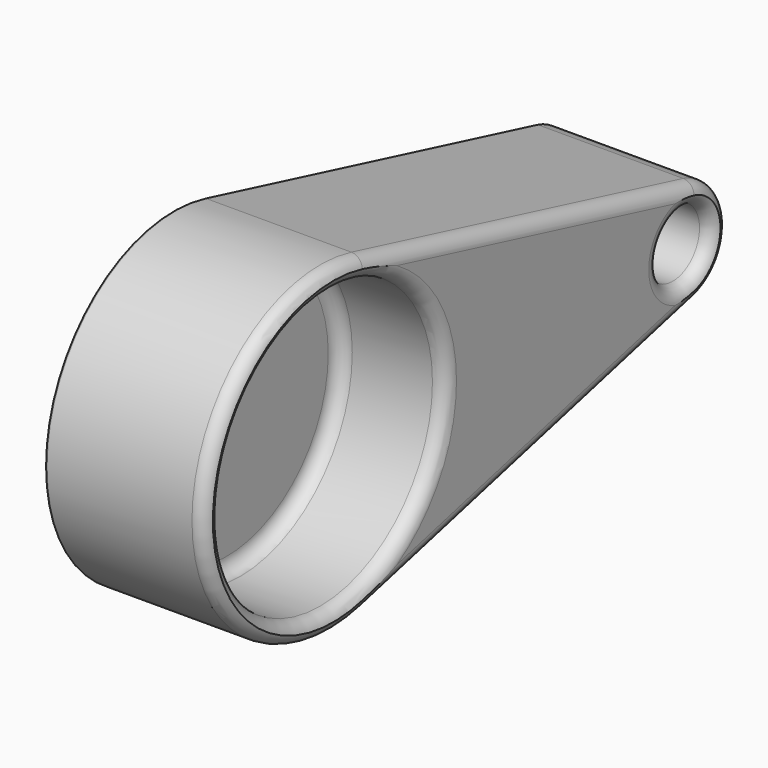
from build123d import *

# Parameters (mm, degrees)
F1_DEPTH = 76.2
F2_R     = 66.675
F2_R_2   = 15.875
F3_DEPTH = 50.8
F4_F1_R  = 6.35
F4_F2_R  = 6.35
F4_F3_R  = 6.35
F5_T     = -2.54
F6_R     = 1


# Not quite as in the source:
# - a fillet or chamfer that OpenCascade refuses, or shapes differently, is made with other operations: its cross-section is extruded or revolved along the edge and cut away or added


with BuildPart() as f1:
    # F0 (on Right) → F1 (new body)
    with BuildSketch(Plane.YZ):
        with BuildLine():
            ThreePointArc((18.4812146278, -73.9248585111), (60.0612543768, -46.8944103565), (76.2, 0))
            ThreePointArc((76.2, 0), (60.0612543768, 46.8944103565), (18.4812146278, 73.9248585111))
            ThreePointArc((18.4812146278, 73.9248585111), (-76.2, 0), (18.4812146278, -73.9248585111))
        make_face()
        with BuildLine():
            ThreePointArc((18.4812146278, 73.9248585111), (60.0612543768, 46.8944103565), (76.2, 0))
            ThreePointArc((76.2, 0), (60.0612543768, -46.8944103565), (18.4812146278, -73.9248585111))
            Line((18.4812146278, -73.9248585111), (215.6141706573, -24.6416195037))
            ThreePointArc((215.6141706573, -24.6416195037), (184.0537657814, 0), (215.6141706573, 24.6416195037))
            Line((215.6141706573, 24.6416195037), (18.4812146278, 73.9248585111))
        make_face()
        with BuildLine():
            ThreePointArc((234.8537657814, 0), (229.474183907, 15.6314701188), (215.6141706573, 24.6416195037))
            ThreePointArc((215.6141706573, 24.6416195037), (184.0537657814, 0), (215.6141706573, -24.6416195037))
            ThreePointArc((215.6141706573, -24.6416195037), (229.474183907, -15.6314701188), (234.8537657814, 0))
        make_face()
    extrude(amount=F1_DEPTH)

    # F2 (on face) → F3 (cut)
    with BuildSketch(Plane.YZ.offset(76.2)):
        Circle(F2_R)
        with Locations((209.4537657814, 0)):
            Circle(F2_R_2)
    extrude(amount=-F3_DEPTH, mode=Mode.SUBTRACT)

    # F4: fillet of radius 6.35 on 8 edges, made by hand

    # F4_f1
    f4_f1_edges = [f1.edges().sort_by_distance(p)[0] for p in [
        (76.2, -76.2, 0),
        (76.2, 117.0476926425, 49.2832390074),
        (76.2, 117.0476926425, -49.2832390074),
        (76.2, 234.8537657814, 0),
    ]]
    fillet(f4_f1_edges, radius=F4_F1_R)

    # F4_f2
    f4_f2_edges = [f1.edges().sort_by_distance(p)[0] for p in [
        (25.4, -66.675, 0),
    ]]
    fillet(f4_f2_edges, radius=F4_F2_R)

    # F4_f3
    f4_f3_edges = [f1.edges().sort_by_distance(p)[0] for p in [
        (25.4, 193.5787657814, 0),
    ]]
    fillet(f4_f3_edges, radius=F4_F3_R)

    # F4_s4 → F4_t5 (revolve, cut)
    with BuildSketch(Plane.XY):
        with BuildLine():
            ThreePointArc((76.2, 73.025), (74.3401280605, 68.5348719395), (69.85, 66.675))
            Line((69.85, 66.675), (69.85, 66.548))
            Line((69.85, 66.548), (76.327, 66.548))
            Line((76.327, 66.548), (76.327, 73.025))
            Line((76.327, 73.025), (76.2, 73.025))
        make_face()
    revolve(axis=Axis((76.2, 0, 0), (1, 0, 0)), mode=Mode.SUBTRACT)

    # F4_s6 → F4_t7 (revolve, cut)
    with BuildSketch(Plane.XY):
        with BuildLine():
            ThreePointArc((69.85, 225.3287657814), (74.3401280605, 227.1886377208), (76.2, 231.6787657814))
            Line((76.2, 231.6787657814), (76.327, 231.6787657814))
            Line((76.327, 231.6787657814), (76.327, 225.2017657814))
            Line((76.327, 225.2017657814), (69.85, 225.2017657814))
            Line((69.85, 225.2017657814), (69.85, 225.3287657814))
        make_face()
    revolve(axis=Axis((76.2, 209.4537657814, 0), (1, 0, 0)), mode=Mode.SUBTRACT)

    # F5
    f5_openings = [f1.faces().sort_by_distance(p)[0] for p in [
        (0, 57.51924, 0),
    ]]
    offset(amount=F5_T, openings=f5_openings)

    # F6
    f6_edges = [f1.edges().sort_by_distance(p)[0] for p in [
        (0, 117.047693, -49.283239),
        (0, 116.431652, -46.819077),
        (0, -76.2, 0),
        (0, -73.66, 0),
        (0, 116.431652, 46.819077),
        (0, 117.047693, 49.283239),
        (0, 232.313766, 0),
        (0, 234.853766, 0),
    ]]
    fillet(f6_edges, radius=F6_R)


solid = f1.part
